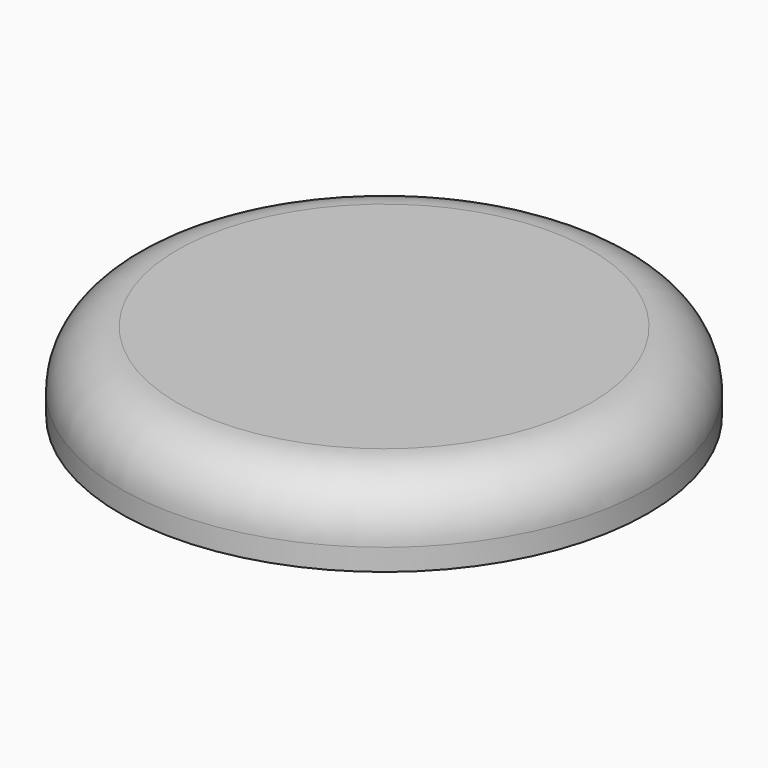
from build123d import *

# Parameters (mm, degrees)
F0_R     = 3.125
F0_R_2   = 1.5
F1_DEPTH = 2.375
F2_R     = 13.4045840815
F2_R_2   = 3.125
F2_R_3   = 1.5
F3_DEPTH = 4
F4_R     = 2.8970562748
F5_R     = 3.85
F5_R_2   = 1.5
F6_DEPTH = 1
F7_DEPTH = 4


with BuildPart() as f1:
    # F0 (on Top) → F1 (new body)
    with BuildSketch(Plane.XY):
        Circle(F0_R)
        Circle(F0_R_2, mode=Mode.SUBTRACT)
    extrude(amount=F1_DEPTH)


with BuildPart() as f3:
    # F2 (on face) → F3 (new body)
    with BuildSketch(Plane.XY.offset(2.375)):
        Circle(F2_R)
        Circle(F2_R_2, mode=Mode.SUBTRACT)
        Circle(F2_R_2)
        Circle(F2_R_3, mode=Mode.SUBTRACT)
    extrude(amount=F3_DEPTH)

    # F4
    f4_edges = [f3.edges().sort_by_distance(p)[0] for p in [
        (-13.404584, 0, 6.375),
    ]]
    fillet(f4_edges, radius=F4_R)

    # F5 (on face) → F7 (join)
    with BuildSketch(Plane(origin=(0, 0, 2.375), x_dir=(1, 0, 0), z_dir=(0, 0, -1))):
        Circle(F5_R)
        Circle(F5_R_2, mode=Mode.SUBTRACT)
        Circle(F5_R_2)
    extrude(amount=-F7_DEPTH)


with BuildPart() as f6:
    # F5 (on face) → F6 (new body)
    with BuildSketch(Plane(origin=(0, 0, 2.375), x_dir=(1, 0, 0), z_dir=(0, 0, -1))):
        Circle(F5_R)
        Circle(F5_R_2, mode=Mode.SUBTRACT)
    extrude(amount=F6_DEPTH)


solid = Compound([f1.part, f3.part, f6.part])
